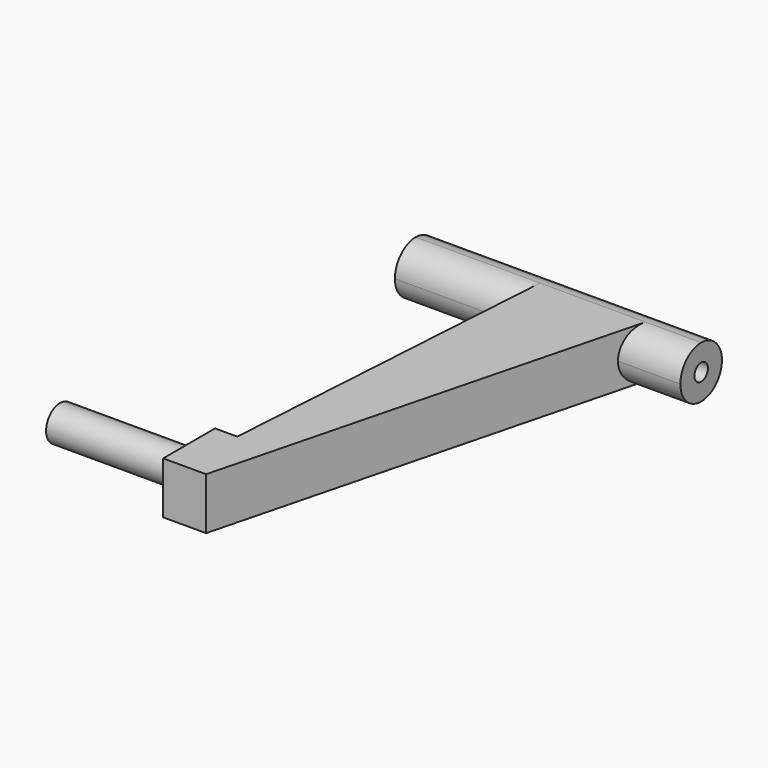
from build123d import *

# Parameters (mm, degrees)
F1_DEPTH = 40
F2_R     = 19.99999
F3_R     = 6.5
F4_DEPTH = 220.001
F5_R     = 13.52259159
F6_DEPTH = 100


# Not quite as in the source:
# - a fillet or chamfer is up to 0.001 mm smaller than in the source, because OpenCascade refuses the exact size


with BuildPart() as f1:
    # F0 (on Top) → F1 (new body)
    with BuildSketch(Plane.XY):
        Polygon((125.4761886686, 235.2380912917), (-94.5238113314, 235.2380912917), (-94.5238113314, 195.2380912917), (0, 195.2380912917), (-15.9523813939, -54.7619087083), (-33.0952398201, -54.7619087083), (-33.0952398201, -104.7619087083), (0, -104.7619087083), (77.3809560928, 195.2380912917), (125.4761886686, 195.2380912917), align=None)
    extrude(amount=F1_DEPTH)

    # F2 (radius 20 in the source; OpenCascade refuses exactly that, so slightly less here)
    f2_edges = [f1.edges().sort_by_distance(p)[0] for p in [
        (15.476189, 235.238091, 40),
        (15.476189, 235.238091, 0),
        (-47.261906, 195.238091, 0),
        (-47.261906, 195.238091, 40),
        (101.428572, 195.238091, 0),
        (101.428572, 195.238091, 40),
    ]]
    fillet(f2_edges, radius=F2_R)

    # F3 (on face) → F4 (cut, through all)
    with BuildSketch(Plane(origin=(-94.5238113314, 0, 0), x_dir=(0, -1, 0), z_dir=(-1, 0, 0))):
        with Locations((-215.2380912917, 20)):
            Circle(F3_R)
    extrude(amount=-F4_DEPTH, mode=Mode.SUBTRACT)

    # F5 (on face) → F6 (join)
    with BuildSketch(Plane(origin=(-33.0952398201, 0, 0), x_dir=(0, -1, 0), z_dir=(-1, 0, 0))):
        with Locations((78.9996907115, 21.1079698056)):
            Circle(F5_R)
    extrude(amount=F6_DEPTH)


solid = f1.part
